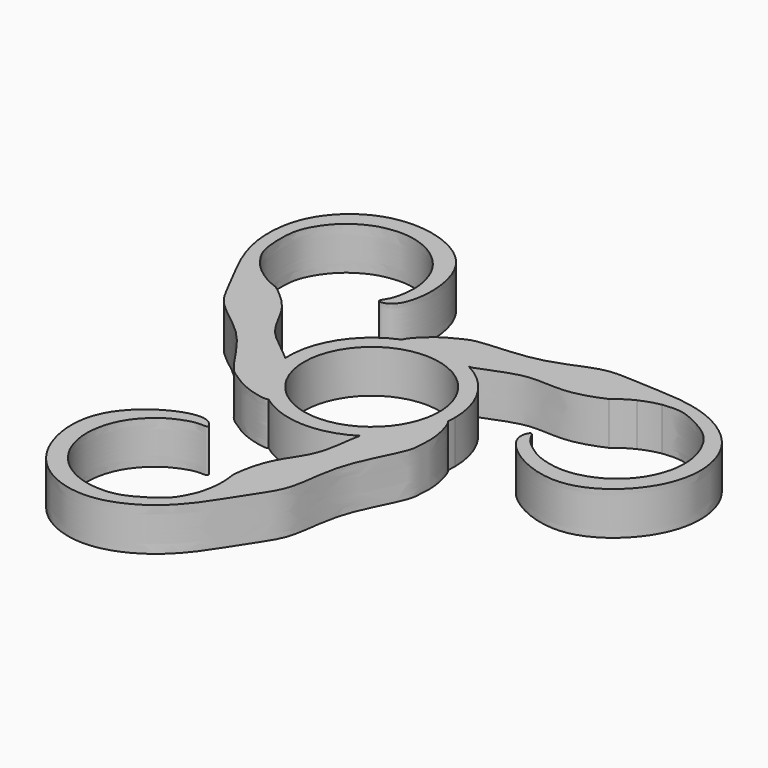
from build123d import *

# Parameters (mm, degrees)
F0_R     = 11
F1_DEPTH = 7
F2_D     = 22


with BuildPart() as f1:
    # F0 (on Top) → F1 (new body)
    with BuildSketch(Plane.XY):
        with BuildLine():
            ThreePointArc((13.4819568605, -1.3844984495), (13.535122126, -0.6931563894), (13.5528593568, 0))
            ThreePointArc((13.5528593568, 0), (11.5409392226, 7.1054006647), (6.1025173623, 12.1012097985))
            ThreePointArc((6.1025173623, 12.1012097985), (5.4286418969, 12.4181256195), (4.7383769517, 12.6975501814))
            add(Edge.make_bspline(
                [(1.4616234128, 13.4738136303), (1.7123979801, 13.086391174), (3.5057767674, 12.9174506871), (4.7383769517, 12.6975501814)],
                knots=[0.8867730843, 0.8867730843, 0.8867730843, 0.8867730843, 0.9749329021, 0.9749329021, 0.9749329021, 0.9749329021], degree=3))
            ThreePointArc((1.4616234128, 13.4738136303), (1.2188934575, 13.4979367121), (0.975768664, 13.5176873858))
            add(Edge.make_bspline(
                [(-5.100113131, 12.5566254542), (-5.1035389964, 12.5334715149), (-5.1587363161, 11.7570033516), (-2.7809338395, 12.561708759), (0.975768664, 13.5176873858)],
                knots=[0.9644549691, 0.9644549691, 0.9644549691, 0.9644549691, 0.9654216454, 0.9986339578, 0.9986339578, 0.9986339578, 0.9986339578], degree=3))
            ThreePointArc((-5.100113131, 12.5566254542), (-11.4368638013, 7.2717359093), (-13.5343244846, -0.7085601529))
            add(Edge.make_bspline(
                [(-13.5121162546, -0.7453970701), (-13.5188089301, -0.7334229075), (-13.5262174696, -0.7211424332), (-13.5343244846, -0.7085601529)],
                knots=[0.0560478924, 0.0560478924, 0.0560478924, 0.0560478924, 0.0586326072, 0.0586326072, 0.0586326072, 0.0586326072], degree=3))
            Line((-13.5121162546, -0.7453970701), (-13.5009697648, -0.7663526387))
            add(Edge.make_bspline(
                [(-13.4924463721, -1.2782361449), (-13.4782795602, -1.0536214618), (-13.4127962108, -0.9411524135), (-13.5009697648, -0.7663526387)],
                knots=[0.0156674938, 0.0156674938, 0.0156674938, 0.0156674938, 0.0545176783, 0.0545176783, 0.0545176783, 0.0545176783], degree=3))
            ThreePointArc((-13.4924463721, -1.2782361449), (-13.4661197601, -1.5308871129), (-13.4350625868, -1.7830002901))
            add(Edge.make_bspline(
                [(-12.278397927, -5.7376773255), (-11.9196723927, -5.3425347034), (-13.1546137837, -2.9093216764), (-13.4350625868, -1.7830002901)],
                knots=[0.8833990224, 0.8833990224, 0.8833990224, 0.8833990224, 0.9941568852, 0.9941568852, 0.9941568852, 0.9941568852], degree=3))
            ThreePointArc((-12.278397927, -5.7376773255), (-12.2019823374, -5.898442488), (-12.1234619071, -6.0581901698))
            add(Edge.make_bspline(
                [(-8.0896676744, -10.8736964122), (-7.5565025003, -10.4715208513), (-9.415271435, -8.8408859982), (-12.1234619071, -6.0581901698)],
                knots=[0.9659212752, 0.9659212752, 0.9659212752, 0.9659212752, 0.9989537493, 0.9989537493, 0.9989537493, 0.9989537493], degree=3))
            ThreePointArc((-8.0896676744, -10.8736964122), (-0.5111727849, -13.5432159818), (7.2469893216, -11.4525605223))
            add(Edge.make_bspline(
                [(8.1096871116, -10.6495548378), (7.7242775111, -10.9729529777), (7.4683993872, -10.8318437649), (7.2868750695, -11.3111197506), (7.2469893216, -11.4525605223)],
                knots=[0, 0, 0, 0, 0.0560478924, 0.0732187107, 0.0732187107, 0.0732187107, 0.0732187107], degree=3))
            add(Edge.make_bspline(
                [(11.1807226284, -7.6204053418), (10.7622890174, -7.0759375914), (8.9670313027, -9.9301552267), (8.1096871116, -10.6495548378)],
                knots=[0.8753213855, 0.8753213855, 0.8753213855, 0.8753213855, 1, 1, 1, 1], degree=3))
            add(Edge.make_bspline(
                [(13.4819568605, -1.3844984495), (13.4760382683, -1.3807535555), (12.8207051619, -0.9920568464), (12.3246594665, -3.6232877277), (11.1807226284, -7.6204053418)],
                knots=[0.9651071634, 0.9651071634, 0.9651071634, 0.9651071634, 0.9654216454, 1, 1, 1, 1], degree=3))
        make_face()
        Circle(F0_R, mode=Mode.SUBTRACT)
        Circle(F0_R)
        with BuildLine():
            add(Edge.make_bspline(
                [(0.8151933987, -36.7336272001), (-0.08204248, -38.7592185172), (-1.0689270281, -40.2000214552), (-6.0950927526, -43.4370960652), (-9.3045918338, -43.5502748302), (-11.1391615138, -43.4016852374), (-12.7894180452, -42.9900074457), (-14.4279393888, -42.3320150023), (-16.2018563655, -41.1578313482), (-17.3706191329, -40.1017807563), (-18.9780278091, -38.0492734337), (-19.9965339763, -35.6172410632), (-20.5253505111, -32.6266556974), (-19.9507292449, -28.9412882739), (-18.4252064579, -25.9992954722), (-16.1649714588, -23.7742388386), (-14.4940492053, -22.7030844288), (-11.3050134017, -21.3418117863), (-8.9114342832, -21.9125827936), (-10.7654704919, -19.2759649055), (-17.0876723558, -20.9279921676), (-23.6099766173, -27.2098699657), (-23.3394838269, -36.0344650137), (-19.7424517516, -42.3214248858), (-14.6073200015, -45.6171562065), (-8.4478817898, -46.4527242335), (-1.8778281579, -43.7339785083), (2.8806701115, -38.7459664101), (6.3086610038, -32.7525612488), (9.8339325466, -28.187440824), (9.7557983337, -19.4196926338), (14.840668149, -11.0617645231), (14.8157101933, -8.493925922), (15.1314493126, -5.744683495), (14.0003730528, -1.7125179613), (13.4819568605, -1.3844984495)],
                knots=[0.0745372635, 0.0745372635, 0.0745372635, 0.0745372635, 0.1023739811, 0.1335381035, 0.1574738716, 0.1753108489, 0.1925093481, 0.2104628232, 0.2297668519, 0.2467130826, 0.2680270009, 0.2898416127, 0.3130586955, 0.3387441591, 0.363309304, 0.3865944457, 0.4058304694, 0.4311179736, 0.4477799897, 0.4651964581, 0.4978590843, 0.5375154795, 0.5758793322, 0.611361041, 0.6436991826, 0.6763707261, 0.7113916566, 0.7465806052, 0.7815871349, 0.8129202034, 0.8526345809, 0.8938291602, 0.9142047732, 0.9375613267, 0.9651071634, 0.9651071634, 0.9651071634, 0.9651071634], degree=3))
            ThreePointArc((13.4819568605, -1.3844984495), (12.7283713279, -4.6549500624), (11.1942482831, -7.6399477827))
            add(Edge.make_bspline(
                [(2.1159909238, -33.6174758818), (4.4965991899, -32.0709896186), (12.169499658, -9.1997897735), (11.1942482831, -7.6399477827)],
                knots=[0.5603344177, 0.5603344177, 0.5603344177, 0.5603344177, 0.8739267879, 0.8739267879, 0.8739267879, 0.8739267879], degree=3))
            add(Edge.make_bspline(
                [(2.1159909238, -33.6174758818), (1.6243927459, -34.8442261783), (1.1834402513, -35.9022765545), (0.8151933987, -36.7336272001)],
                knots=[0.0631124154, 0.0631124154, 0.0631124154, 0.0631124154, 0.0745372635, 0.0745372635, 0.0745372635, 0.0745372635], degree=3))
        make_face()
        with BuildLine():
            Line((-8.115507743, -10.8911022488), (-8.1479656373, -10.8300809194))
            ThreePointArc((-8.1479656373, -10.8300809194), (-10.4127531903, -8.6749390628), (-12.1234619071, -6.0581901698))
            add(Edge.make_bspline(
                [(-12.1234619071, -6.0581901698), (-12.2092395023, -5.9700527367), (-12.2958692408, -5.8807595513), (-12.3833021093, -5.7903130411)],
                knots=[0.9989537493, 0.9989537493, 0.9989537493, 0.9989537493, 1, 1, 1, 1], degree=3))
            add(Edge.make_bspline(
                [(-30.3650597686, 15.0585101635), (-30.2154049176, 12.210992477), (-14.1031169928, -6.0180426147), (-12.3833021093, -5.7903130411)],
                knots=[0.5603344177, 0.5603344177, 0.5603344177, 0.5603344177, 0.8753213855, 0.8753213855, 0.8753213855, 0.8753213855], degree=3))
            add(Edge.make_bspline(
                [(-30.3650597686, 15.0585101635), (-31.1816576006, 16.0976218223), (-31.8774798575, 17.0085230726), (-32.4133272097, 17.7431095246)],
                knots=[0.0631124154, 0.0631124154, 0.0631124154, 0.0631124154, 0.0745372635, 0.0745372635, 0.0745372635, 0.0745372635], degree=3))
            add(Edge.make_bspline(
                [(-32.4133272097, 17.7431095246), (-33.7189228087, 19.5329342473), (-34.4732524808, 21.1080028055), (-34.7635584648, 27.0793273116), (-33.2568246098, 29.9154244319), (-32.2108574077, 31.4299135834), (-31.0292057163, 32.6532387665), (-29.6401068729, 33.743243653), (-27.7362755114, 34.6924089919), (-26.2373274875, 35.1765619436), (-23.6560996665, 35.5423650302), (-21.0406447672, 35.2084010595), (-18.1863136009, 34.1710769297), (-15.282002423, 31.8307566039), (-13.4969233125, 29.0386187155), (-12.7000852424, 25.968669471), (-12.6078994389, 23.9860311467), (-13.0235206508, 20.543608806), (-14.7146124022, 18.7560939871), (-11.5042162267, 19.0434274993), (-9.7738128714, 25.3446285523), (-11.9529264972, 34.134048633), (-19.7304963822, 38.312092529), (-26.9736793816, 38.3404513097), (-32.3954323045, 35.5411624226), (-36.1987745483, 30.6247164717), (-37.1292984998, 23.5755102597), (-35.1888024431, 16.9605238254), (-31.7123567643, 10.9950940481), (-29.5214822765, 5.6595591244), (-21.8893225034, 1.3433512426), (-17.1935793441, -7.2392392478), (-14.957286905, -8.5015443246), (-12.7244345021, -10.1568749545), (-8.6265170015, -11.1989480561), (-8.1155077304, -10.8911022412)],
                knots=[0.0745372635, 0.0745372635, 0.0745372635, 0.0745372635, 0.1023739811, 0.1335381035, 0.1574738716, 0.1753108489, 0.1925093481, 0.2104628232, 0.2297668519, 0.2467130826, 0.2680270009, 0.2898416127, 0.3130586955, 0.3387441591, 0.363309304, 0.3865944457, 0.4058304694, 0.4311179736, 0.4477799897, 0.4651964581, 0.4978590843, 0.5375154795, 0.5758793322, 0.611361041, 0.6436991826, 0.6763707261, 0.7113916566, 0.7465806052, 0.7815871349, 0.8129202034, 0.8526345809, 0.8938291602, 0.9142047732, 0.9375613267, 0.9654216454, 0.9654216454, 0.9654216454, 0.9654216454], degree=3))
        make_face()
        with BuildLine():
            ThreePointArc((-5.100113131, 12.5566254542), (-2.1174192617, 13.3864309066), (0.975768664, 13.5176873858))
            add(Edge.make_bspline(
                [(0.975768664, 13.5176873858), (1.1302840758, 13.5570073562), (1.2872459785, 13.5966217419), (1.4465951461, 13.636438767)],
                knots=[0.9986339578, 0.9986339578, 0.9986339578, 0.9986339578, 1, 1, 1, 1], degree=3))
            add(Edge.make_bspline(
                [(28.49308451, 18.7846861024), (25.9522344302, 20.0788400429), (2.1092829919, 15.2397069328), (1.4465951461, 13.636438767)],
                knots=[0.5603344177, 0.5603344177, 0.5603344177, 0.5603344177, 0.8753213855, 0.8753213855, 0.8753213855, 0.8753213855], degree=3))
            add(Edge.make_bspline(
                [(28.49308451, 18.7846861024), (29.8012805198, 18.9723247402), (30.9380552714, 19.119473866), (31.8421494762, 19.2162380596)],
                knots=[0.0631124154, 0.0631124154, 0.0631124154, 0.0631124154, 0.0745372635, 0.0745372635, 0.0745372635, 0.0745372635], degree=3))
            add(Edge.make_bspline(
                [(31.8421494762, 19.2162380596), (34.0449809539, 19.452004654), (35.7861951741, 19.3177390338), (41.1026668825, 16.5834891378), (42.8054321088, 13.8605707824), (43.5940345867, 12.1974920382), (44.0626394266, 10.5624890634), (44.312061927, 8.8144917335), (44.1821475421, 6.6911427404), (43.8519622856, 5.1509391969), (42.8781431409, 2.7326287877), (41.2811944087, 0.6345603878), (38.9556797771, -1.3187008482), (35.476747333, -2.6637479458), (32.1661454356, -2.8136028591), (29.1090723665, -1.9687102482), (27.3459643093, -1.0572263338), (24.5725497177, 1.0239233644), (23.8700623506, 3.3822091907), (22.5137023837, 0.4582577904), (27.1055008924, -4.1909160006), (35.8069187797, -6.6984582832), (43.3139958742, -2.0519071312), (46.9601467985, 4.2066939603), (47.2467679711, 10.3017141681), (44.8906720032, 16.0537281459), (39.2511423229, 20.3841886328), (32.5521479967, 22.0111629689), (25.6477114257, 21.9831875848), (19.9315653951, 22.7536020837), (12.3775398349, 18.3020617753), (2.5969268603, 18.526724155), (0.3855923769, 17.2211906308), (-2.12996108, 16.130083349), (-5.0048030456, 13.2007850196), (-5.100113131, 12.5566254542)],
                knots=[0.0745372635, 0.0745372635, 0.0745372635, 0.0745372635, 0.1023739811, 0.1335381035, 0.1574738716, 0.1753108489, 0.1925093481, 0.2104628232, 0.2297668519, 0.2467130826, 0.2680270009, 0.2898416127, 0.3130586955, 0.3387441591, 0.363309304, 0.3865944457, 0.4058304694, 0.4311179736, 0.4477799897, 0.4651964581, 0.4978590843, 0.5375154795, 0.5758793322, 0.611361041, 0.6436991826, 0.6763707261, 0.7113916566, 0.7465806052, 0.7815871349, 0.8129202034, 0.8526345809, 0.8938291602, 0.9142047732, 0.9375613267, 0.9644549691, 0.9644549691, 0.9644549691, 0.9644549691], degree=3))
        make_face()
        with BuildLine():
            ThreePointArc((1.4616234128, 13.4738136303), (3.124203477, 13.1878485501), (4.7383769517, 12.6975501814))
            add(Edge.make_bspline(
                [(4.7383769517, 12.6975501814), (5.0888507865, 12.635024332), (5.3939870575, 12.5683784911), (5.6054333199, 12.4914187415)],
                knots=[0.9749329021, 0.9749329021, 0.9749329021, 0.9749329021, 1, 1, 1, 1], degree=3))
            add(Edge.make_bspline(
                [(5.6054333199, 12.4914187415), (6.0653014484, 12.3240412925), (6.0820102677, 12.1078784425), (6.3563063141, 12.0923871482)],
                knots=[0, 0, 0, 0, 0.0545176786, 0.0545176786, 0.0545176786, 0.0545176786], degree=3))
            add(Edge.make_bspline(
                [(6.3563063141, 12.0923871482), (6.3640053139, 12.0919523353), (6.3719072472, 12.0916756163), (6.3800276096, 12.0915625076)],
                knots=[0.0545176786, 0.0545176786, 0.0545176786, 0.0545176786, 0.0560478924, 0.0560478924, 0.0560478924, 0.0560478924], degree=3))
            add(Edge.make_bspline(
                [(6.3800276096, 12.0915625076), (7.2290913033, 12.0797358729), (14.0523207762, 15.8250954038), (18.9510522497, 13.7009373073), (24.4062863921, 15.6672470824), (25.6121017726, 16.2173204292)],
                knots=[0.0560478924, 0.0560478924, 0.0560478924, 0.0560478924, 0.2160467846, 0.3932975033, 0.4533339453, 0.4533339453, 0.4533339453, 0.4533339453], degree=3))
            ThreePointArc((25.6121017726, 16.2173204292), (27.055447812, 17.3016603109), (28.6327278696, 18.1798564099))
            add(Edge.make_bspline(
                [(28.6327278696, 18.1798564099), (28.7933733657, 18.4341528484), (28.7671438841, 18.6450969855), (28.49308451, 18.7846861024)],
                knots=[0.5263595162, 0.5263595162, 0.5263595162, 0.5263595162, 0.5603344177, 0.5603344177, 0.5603344177, 0.5603344177], degree=3))
            add(Edge.make_bspline(
                [(1.4465951461, 13.636438767), (8.8086743733, 15.4760222302), (21.2664317766, 17.7481447399), (28.49308451, 18.7846861024)],
                knots=[0, 0, 0, 0, 0.0631124154, 0.0631124154, 0.0631124154, 0.0631124154], degree=3))
            add(Edge.make_bspline(
                [(1.4465951461, 13.636438767), (1.4225023983, 13.5781501839), (1.4290485406, 13.5241386579), (1.4616234128, 13.4738136303)],
                knots=[0.8753213855, 0.8753213855, 0.8753213855, 0.8753213855, 0.8867730843, 0.8867730843, 0.8867730843, 0.8867730843], degree=3))
        make_face()
        with BuildLine():
            ThreePointArc((-13.4924463721, -1.2782361449), (-13.5163870328, -0.9936188033), (-13.5343244846, -0.7085601529))
            add(Edge.make_bspline(
                [(-13.5343244846, -0.7085601529), (-14.0280575297, 0.0577252822), (-20.5855644279, 4.0667480011), (-21.1913880355, 9.33674222), (-25.6218793236, 13.0779586833), (-26.7011645061, 13.8471887617)],
                knots=[0.0586326072, 0.0586326072, 0.0586326072, 0.0586326072, 0.2160467846, 0.3932975033, 0.4533339453, 0.4533339453, 0.4533339453, 0.4533339453], degree=3))
            ThreePointArc((-26.7011645061, 13.8471887617), (-28.3619034097, 14.5549931574), (-29.9110835698, 15.4818597067))
            add(Edge.make_bspline(
                [(-29.9110835698, 15.4818597067), (-30.2116334936, 15.4938345681), (-30.3812017343, 15.3656471022), (-30.3650597686, 15.0585101635)],
                knots=[0.5263595162, 0.5263595162, 0.5263595162, 0.5263595162, 0.5603344177, 0.5603344177, 0.5603344177, 0.5603344177], degree=3))
            add(Edge.make_bspline(
                [(-12.3833021093, -5.7903130411), (-17.6574677344, -0.3343571373), (-25.85406225, 9.3183159934), (-30.3650597686, 15.0585101635)],
                knots=[0, 0, 0, 0, 0.0631124154, 0.0631124154, 0.0631124154, 0.0631124154], degree=3))
            add(Edge.make_bspline(
                [(-12.3833021093, -5.7903130411), (-12.3391985702, -5.7844730636), (-12.3045599937, -5.766495312), (-12.278397927, -5.7376773255)],
                knots=[0.8753213855, 0.8753213855, 0.8753213855, 0.8753213855, 0.8833990224, 0.8833990224, 0.8833990224, 0.8833990224], degree=3))
            ThreePointArc((-12.278397927, -5.7376773255), (-13.007896852, -3.8045520411), (-13.4350625868, -1.7830002901))
            add(Edge.make_bspline(
                [(-13.4350625868, -1.7830002901), (-13.4498578755, -1.7235803536), (-13.4619966492, -1.6677977185), (-13.4711047662, -1.6161435196)],
                knots=[0.9941568852, 0.9941568852, 0.9941568852, 0.9941568852, 1, 1, 1, 1], degree=3))
            add(Edge.make_bspline(
                [(-13.4711047662, -1.6161435196), (-13.4955269061, -1.4776400217), (-13.4981595608, -1.3688187043), (-13.4924463721, -1.2782361449)],
                knots=[0, 0, 0, 0, 0.0156674938, 0.0156674938, 0.0156674938, 0.0156674938], degree=3))
        make_face()
        with BuildLine():
            add(Edge.make_bspline(
                [(11.1613906196, -7.6878707184), (9.0666047055, -14.9892692887), (4.8232914209, -26.8615889868), (2.1159909238, -33.6174758818)],
                knots=[0.0001941654, 0.0001941654, 0.0001941654, 0.0001941654, 0.0631124154, 0.0631124154, 0.0631124154, 0.0631124154], degree=3))
            ThreePointArc((11.1613906196, -7.6878707184), (9.3946971928, -9.7682987977), (7.2469893216, -11.4525605223))
            add(Edge.make_bspline(
                [(7.2469893216, -11.4525605223), (6.9152168671, -12.6290748039), (6.587922805, -19.7690678016), (2.484351451, -22.8119591431), (1.4596085967, -28.5194853816), (1.3330783987, -29.8387888067)],
                knots=[0.0732187107, 0.0732187107, 0.0732187107, 0.0732187107, 0.2160467846, 0.3932975033, 0.4533339453, 0.4533339453, 0.4533339453, 0.4533339453], degree=3))
            ThreePointArc((1.3330783987, -29.8387888067), (1.5504712629, -31.6309330842), (1.5223713654, -33.4359957324))
            add(Edge.make_bspline(
                [(1.5223713654, -33.4359957324), (1.6622757931, -33.7022670323), (1.8580735154, -33.7850237035), (2.1159909238, -33.6174758818)],
                knots=[0.5263595162, 0.5263595162, 0.5263595162, 0.5263595162, 0.5603344177, 0.5603344177, 0.5603344177, 0.5603344177], degree=3))
        make_face()
        with BuildLine():
            add(Edge.make_bspline(
                [(28.49308451, 18.7846861024), (25.9522344302, 20.0788400429), (2.1092829919, 15.2397069328), (1.4465951461, 13.636438767)],
                knots=[0.5603344177, 0.5603344177, 0.5603344177, 0.5603344177, 0.8753213855, 0.8753213855, 0.8753213855, 0.8753213855], degree=3))
            add(Edge.make_bspline(
                [(1.4465951461, 13.636438767), (8.8086743733, 15.4760222302), (21.2664317766, 17.7481447399), (28.49308451, 18.7846861024)],
                knots=[0, 0, 0, 0, 0.0631124154, 0.0631124154, 0.0631124154, 0.0631124154], degree=3))
        make_face()
        with BuildLine():
            add(Edge.make_bspline(
                [(-30.3650597686, 15.0585101635), (-30.2154049176, 12.210992477), (-14.1031169928, -6.0180426147), (-12.3833021093, -5.7903130411)],
                knots=[0.5603344177, 0.5603344177, 0.5603344177, 0.5603344177, 0.8753213855, 0.8753213855, 0.8753213855, 0.8753213855], degree=3))
            add(Edge.make_bspline(
                [(-12.3833021093, -5.7903130411), (-17.6574677344, -0.3343571373), (-25.85406225, 9.3183159934), (-30.3650597686, 15.0585101635)],
                knots=[0, 0, 0, 0, 0.0631124154, 0.0631124154, 0.0631124154, 0.0631124154], degree=3))
        make_face()
        with BuildLine():
            add(Edge.make_bspline(
                [(2.1159909238, -33.6174758818), (4.4965991899, -32.0709896186), (12.169499658, -9.1997897735), (11.1942482831, -7.6399477827)],
                knots=[0.5603344177, 0.5603344177, 0.5603344177, 0.5603344177, 0.8739267879, 0.8739267879, 0.8739267879, 0.8739267879], degree=3))
            ThreePointArc((11.1942482831, -7.6399477827), (11.1778451339, -7.6639268595), (11.1613906196, -7.6878707184))
            add(Edge.make_bspline(
                [(11.1613906196, -7.6878707184), (9.0666047055, -14.9892692887), (4.8232914209, -26.8615889868), (2.1159909238, -33.6174758818)],
                knots=[0.0001941654, 0.0001941654, 0.0001941654, 0.0001941654, 0.0631124154, 0.0631124154, 0.0631124154, 0.0631124154], degree=3))
        make_face()
        with BuildLine():
            ThreePointArc((11.1942482831, -7.6399477827), (12.7283713279, -4.6549500624), (13.4819568605, -1.3844984495))
            add(Edge.make_bspline(
                [(13.4819568605, -1.3844984495), (13.4760382683, -1.3807535555), (12.8207051619, -0.9920568464), (12.3246594665, -3.6232877277), (11.1807226284, -7.6204053418)],
                knots=[0.9651071634, 0.9651071634, 0.9651071634, 0.9651071634, 0.9654216454, 1, 1, 1, 1], degree=3))
            add(Edge.make_bspline(
                [(11.1942482831, -7.6399477827), (11.1899111773, -7.6330109048), (11.1854030344, -7.6264955078), (11.1807226284, -7.6204053418)],
                knots=[0.8739267879, 0.8739267879, 0.8739267879, 0.8739267879, 0.8753213855, 0.8753213855, 0.8753213855, 0.8753213855], degree=3))
        make_face()
        with BuildLine():
            add(Edge.make_bspline(
                [(-5.100113131, 12.5566254542), (-5.1035389964, 12.5334715149), (-5.1587363161, 11.7570033516), (-2.7809338395, 12.561708759), (0.975768664, 13.5176873858)],
                knots=[0.9644549691, 0.9644549691, 0.9644549691, 0.9644549691, 0.9654216454, 0.9986339578, 0.9986339578, 0.9986339578, 0.9986339578], degree=3))
            ThreePointArc((0.975768664, 13.5176873858), (-2.1174192617, 13.3864309066), (-5.100113131, 12.5566254542))
        make_face()
        with BuildLine():
            ThreePointArc((-8.1479656373, -10.8300809194), (-8.1188459444, -10.8519278138), (-8.0896676744, -10.8736964122))
            add(Edge.make_bspline(
                [(-8.0896676744, -10.8736964122), (-7.5565025003, -10.4715208513), (-9.415271435, -8.8408859982), (-12.1234619071, -6.0581901698)],
                knots=[0.9659212752, 0.9659212752, 0.9659212752, 0.9659212752, 0.9989537493, 0.9989537493, 0.9989537493, 0.9989537493], degree=3))
            ThreePointArc((-12.1234619071, -6.0581901698), (-10.4127531903, -8.6749390628), (-8.1479656373, -10.8300809194))
        make_face()
        with BuildLine():
            add(Edge.make_bspline(
                [(11.1807226284, -7.6204053418), (11.1742991588, -7.6428500803), (11.1678551198, -7.6653386341), (11.1613906196, -7.6878707184)],
                knots=[0, 0, 0, 0, 0.0001941654, 0.0001941654, 0.0001941654, 0.0001941654], degree=3))
            add(Edge.make_bspline(
                [(11.1807226284, -7.6204053418), (10.7622890174, -7.0759375914), (8.9670313027, -9.9301552267), (8.1096871116, -10.6495548378)],
                knots=[0.8753213855, 0.8753213855, 0.8753213855, 0.8753213855, 1, 1, 1, 1], degree=3))
            add(Edge.make_bspline(
                [(8.1096871116, -10.6495548378), (7.7242775111, -10.9729529777), (7.4683993872, -10.8318437649), (7.2868750695, -11.3111197506), (7.2469893216, -11.4525605223)],
                knots=[0, 0, 0, 0, 0.0560478924, 0.0732187107, 0.0732187107, 0.0732187107, 0.0732187107], degree=3))
            ThreePointArc((7.2469893216, -11.4525605223), (9.3946971928, -9.7682987977), (11.1613906196, -7.6878707184))
        make_face()
        with BuildLine():
            ThreePointArc((-13.4350625868, -1.7830002901), (-13.007896852, -3.8045520411), (-12.278397927, -5.7376773255))
            add(Edge.make_bspline(
                [(-12.278397927, -5.7376773255), (-11.9196723927, -5.3425347034), (-13.1546137837, -2.9093216764), (-13.4350625868, -1.7830002901)],
                knots=[0.8833990224, 0.8833990224, 0.8833990224, 0.8833990224, 0.9941568852, 0.9941568852, 0.9941568852, 0.9941568852], degree=3))
        make_face()
        with BuildLine():
            ThreePointArc((1.5223713654, -33.4359957324), (1.2740741951, -35.1073913243), (0.8151933987, -36.7336272001))
            add(Edge.make_bspline(
                [(2.1159909238, -33.6174758818), (1.6243927459, -34.8442261783), (1.1834402513, -35.9022765545), (0.8151933987, -36.7336272001)],
                knots=[0.0631124154, 0.0631124154, 0.0631124154, 0.0631124154, 0.0745372635, 0.0745372635, 0.0745372635, 0.0745372635], degree=3))
            add(Edge.make_bspline(
                [(1.5223713654, -33.4359957324), (1.6622757931, -33.7022670323), (1.8580735154, -33.7850237035), (2.1159909238, -33.6174758818)],
                knots=[0.5263595162, 0.5263595162, 0.5263595162, 0.5263595162, 0.5603344177, 0.5603344177, 0.5603344177, 0.5603344177], degree=3))
        make_face()
        with BuildLine():
            add(Edge.make_bspline(
                [(28.49308451, 18.7846861024), (29.8012805198, 18.9723247402), (30.9380552714, 19.119473866), (31.8421494762, 19.2162380596)],
                knots=[0.0631124154, 0.0631124154, 0.0631124154, 0.0631124154, 0.0745372635, 0.0745372635, 0.0745372635, 0.0745372635], degree=3))
            add(Edge.make_bspline(
                [(28.6327278696, 18.1798564099), (28.7933733657, 18.4341528484), (28.7671438841, 18.6450969855), (28.49308451, 18.7846861024)],
                knots=[0.5263595162, 0.5263595162, 0.5263595162, 0.5263595162, 0.5603344177, 0.5603344177, 0.5603344177, 0.5603344177], degree=3))
            ThreePointArc((28.6327278696, 18.1798564099), (30.204347497, 18.8005225486), (31.8421494762, 19.2162380596))
        make_face()
        with BuildLine():
            ThreePointArc((-29.9110835698, 15.4818597067), (-31.2344060269, 16.5325891598), (-32.4133272097, 17.7431095246))
            add(Edge.make_bspline(
                [(-30.3650597686, 15.0585101635), (-31.1816576006, 16.0976218223), (-31.8774798575, 17.0085230726), (-32.4133272097, 17.7431095246)],
                knots=[0.0631124154, 0.0631124154, 0.0631124154, 0.0631124154, 0.0745372635, 0.0745372635, 0.0745372635, 0.0745372635], degree=3))
            add(Edge.make_bspline(
                [(-29.9110835698, 15.4818597067), (-30.2116334936, 15.4938345681), (-30.3812017343, 15.3656471022), (-30.3650597686, 15.0585101635)],
                knots=[0.5263595162, 0.5263595162, 0.5263595162, 0.5263595162, 0.5603344177, 0.5603344177, 0.5603344177, 0.5603344177], degree=3))
        make_face()
        with BuildLine():
            add(Edge.make_bspline(
                [(1.4616234128, 13.4738136303), (1.7123979801, 13.086391174), (3.5057767674, 12.9174506871), (4.7383769517, 12.6975501814)],
                knots=[0.8867730843, 0.8867730843, 0.8867730843, 0.8867730843, 0.9749329021, 0.9749329021, 0.9749329021, 0.9749329021], degree=3))
            ThreePointArc((4.7383769517, 12.6975501814), (3.124203477, 13.1878485501), (1.4616234128, 13.4738136303))
        make_face()
        with BuildLine():
            ThreePointArc((4.7383769517, 12.6975501814), (5.4286418969, 12.4181256195), (6.1025173623, 12.1012097985))
            Line((6.1025173623, 12.1012097985), (6.3563063141, 12.0923871482))
            add(Edge.make_bspline(
                [(5.6054333199, 12.4914187415), (6.0653014484, 12.3240412925), (6.0820102677, 12.1078784425), (6.3563063141, 12.0923871482)],
                knots=[0, 0, 0, 0, 0.0545176786, 0.0545176786, 0.0545176786, 0.0545176786], degree=3))
            add(Edge.make_bspline(
                [(4.7383769517, 12.6975501814), (5.0888507865, 12.635024332), (5.3939870575, 12.5683784911), (5.6054333199, 12.4914187415)],
                knots=[0.9749329021, 0.9749329021, 0.9749329021, 0.9749329021, 1, 1, 1, 1], degree=3))
        make_face()
        with BuildLine():
            ThreePointArc((0.975768664, 13.5176873858), (1.2188934575, 13.4979367121), (1.4616234128, 13.4738136303))
            add(Edge.make_bspline(
                [(1.4465951461, 13.636438767), (1.4225023983, 13.5781501839), (1.4290485406, 13.5241386579), (1.4616234128, 13.4738136303)],
                knots=[0.8753213855, 0.8753213855, 0.8753213855, 0.8753213855, 0.8867730843, 0.8867730843, 0.8867730843, 0.8867730843], degree=3))
            add(Edge.make_bspline(
                [(0.975768664, 13.5176873858), (1.1302840758, 13.5570073562), (1.2872459785, 13.5966217419), (1.4465951461, 13.636438767)],
                knots=[0.9986339578, 0.9986339578, 0.9986339578, 0.9986339578, 1, 1, 1, 1], degree=3))
        make_face()
        with BuildLine():
            add(Edge.make_bspline(
                [(-13.5121162546, -0.7453970701), (-13.5188089301, -0.7334229075), (-13.5262174696, -0.7211424332), (-13.5343244846, -0.7085601529)],
                knots=[0.0560478924, 0.0560478924, 0.0560478924, 0.0560478924, 0.0586326072, 0.0586326072, 0.0586326072, 0.0586326072], degree=3))
            ThreePointArc((-13.5343244846, -0.7085601529), (-13.5163870328, -0.9936188033), (-13.4924463721, -1.2782361449))
            add(Edge.make_bspline(
                [(-13.4924463721, -1.2782361449), (-13.4782795602, -1.0536214618), (-13.4127962108, -0.9411524135), (-13.5009697648, -0.7663526387)],
                knots=[0.0156674938, 0.0156674938, 0.0156674938, 0.0156674938, 0.0545176783, 0.0545176783, 0.0545176783, 0.0545176783], degree=3))
            Line((-13.5009697648, -0.7663526387), (-13.5121162546, -0.7453970701))
        make_face()
        with BuildLine():
            add(Edge.make_bspline(
                [(-12.1234619071, -6.0581901698), (-12.2092395023, -5.9700527367), (-12.2958692408, -5.8807595513), (-12.3833021093, -5.7903130411)],
                knots=[0.9989537493, 0.9989537493, 0.9989537493, 0.9989537493, 1, 1, 1, 1], degree=3))
            ThreePointArc((-12.1234619071, -6.0581901698), (-12.2019823374, -5.898442488), (-12.278397927, -5.7376773255))
            add(Edge.make_bspline(
                [(-12.3833021093, -5.7903130411), (-12.3391985702, -5.7844730636), (-12.3045599937, -5.766495312), (-12.278397927, -5.7376773255)],
                knots=[0.8753213855, 0.8753213855, 0.8753213855, 0.8753213855, 0.8833990224, 0.8833990224, 0.8833990224, 0.8833990224], degree=3))
        make_face()
        with BuildLine():
            ThreePointArc((-13.4350625868, -1.7830002901), (-13.4661197601, -1.5308871129), (-13.4924463721, -1.2782361449))
            add(Edge.make_bspline(
                [(-13.4711047662, -1.6161435196), (-13.4955269061, -1.4776400217), (-13.4981595608, -1.3688187043), (-13.4924463721, -1.2782361449)],
                knots=[0, 0, 0, 0, 0.0156674938, 0.0156674938, 0.0156674938, 0.0156674938], degree=3))
            add(Edge.make_bspline(
                [(-13.4350625868, -1.7830002901), (-13.4498578755, -1.7235803536), (-13.4619966492, -1.6677977185), (-13.4711047662, -1.6161435196)],
                knots=[0.9941568852, 0.9941568852, 0.9941568852, 0.9941568852, 1, 1, 1, 1], degree=3))
        make_face()
        with BuildLine():
            ThreePointArc((11.1613906196, -7.6878707184), (11.1778451339, -7.6639268595), (11.1942482831, -7.6399477827))
            add(Edge.make_bspline(
                [(11.1942482831, -7.6399477827), (11.1899111773, -7.6330109048), (11.1854030344, -7.6264955078), (11.1807226284, -7.6204053418)],
                knots=[0.8739267879, 0.8739267879, 0.8739267879, 0.8739267879, 0.8753213855, 0.8753213855, 0.8753213855, 0.8753213855], degree=3))
            add(Edge.make_bspline(
                [(11.1807226284, -7.6204053418), (11.1742991588, -7.6428500803), (11.1678551198, -7.6653386341), (11.1613906196, -7.6878707184)],
                knots=[0, 0, 0, 0, 0.0001941654, 0.0001941654, 0.0001941654, 0.0001941654], degree=3))
        make_face()
    extrude(amount=F1_DEPTH)

    # F2 (through all)
    with Locations(Plane(origin=(0, 0, 0), x_dir=(1, 0, 0), z_dir=(0, 0, -1))):
        with Locations((0, 0)):
            Hole(F2_D / 2)


solid = f1.part
